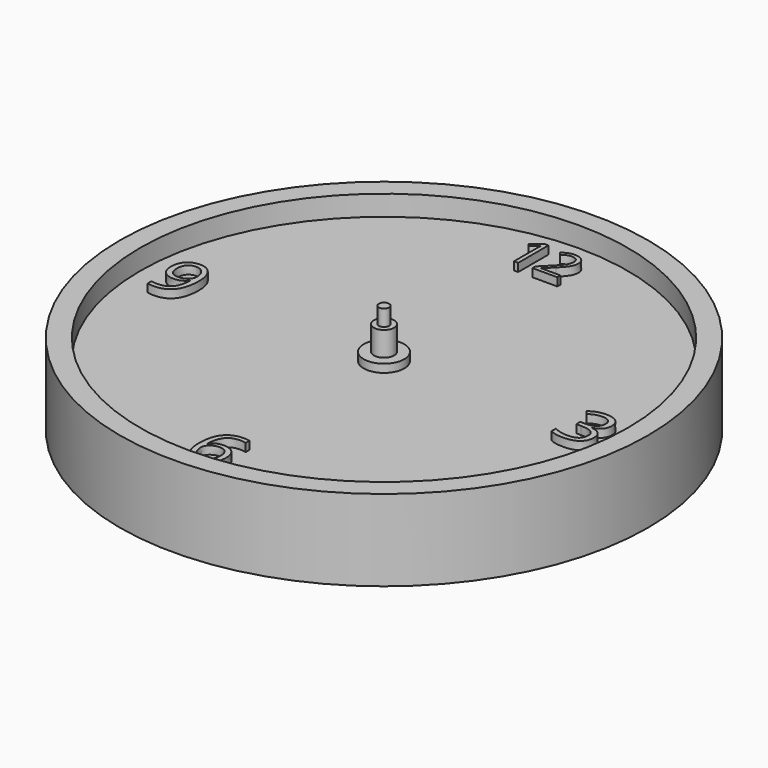
from build123d import *

# Parameters (mm, degrees)
F0_W           = 76.2
F0_H           = 6.35
F3_R           = 6.35
F3_R_2         = 3.175
F3_TEXT_SIZE   = 16.49797023
F3_TEXT_SIZE_2 = 21.9735063531
F3_TEXT_SIZE_3 = 21.605528974
F3_TEXT_SIZE_4 = 21.7850442241
F4_DEPTH       = 2.54
F3_R_3         = 1.5875
F5_DEPTH       = 6.35
F6_DEPTH       = 10.16
F6_DEPTH_BACK  = 12.7
F7_DEPTH       = 15.24
F7_DEPTH_BACK  = 25.4
F8_R           = 3.175
F9_DEPTH       = 6.35
F8_R_2         = 1.8294732505


# Not quite as in the source:
# - Text() gives the source's letters only with a copy of the font that has no kerning and outlines rounded to 1/6400 em; it was checked with that copy


with BuildPart() as f1:
    # F0 (on Front) → F1 (revolve)
    with BuildSketch(Plane.XZ):
        with Locations((-38.1, 3.175)):
            Rectangle(F0_W, F0_H)
    revolve(axis=Axis((0, 0, 3.175), (0, 0, 1)))

    # F3 (on face) → F5 (cut)
    with BuildSketch(Plane.XY.offset(6.35)):
        Circle(F3_R_2)
        Circle(F3_R_3, mode=Mode.SUBTRACT)
        Circle(F3_R_3)
    extrude(amount=-F5_DEPTH, mode=Mode.SUBTRACT)


with BuildPart() as f2:
    # F0 (on Front) → F2 (revolve)
    with BuildSketch(Plane.XZ):
        Polygon((-76.2, -12.7), (-76.2, 0), (-76.2, 6.35), (-76.2, 12.7), (-82.55, 12.7), (-82.55, -12.7), align=None)
    revolve(axis=Axis((0, 0, 3.175), (0, 0, 1)))


with BuildPart() as f4:
    # F3 (on face) → F4 (new body)
    with BuildSketch(Plane.XY.offset(6.35)):
        Circle(F3_R)
        Circle(F3_R_2, mode=Mode.SUBTRACT)
        with Locations((-9.525, 57.15)):
            Text('12', F3_TEXT_SIZE, font='Open Sans', text_align=(TextAlign.LEFT, TextAlign.BOTTOM))
        with Locations((57.15, -7.9104622871)):
            Text('3', F3_TEXT_SIZE_2, font='Open Sans', text_align=(TextAlign.LEFT, TextAlign.BOTTOM))
        with Locations((-6.35, -72.7059808612)):
            Text('6', F3_TEXT_SIZE_3, font='Open Sans', text_align=(TextAlign.LEFT, TextAlign.BOTTOM))
        with Locations((-69.85, -7.8426159207)):
            Text('9', F3_TEXT_SIZE_4, font='Open Sans', text_align=(TextAlign.LEFT, TextAlign.BOTTOM))
    extrude(amount=F4_DEPTH)


with BuildPart() as f6:
    # F3 (on face) → F6 (new body, two sides)
    with BuildSketch(Plane.XY.offset(6.35)) as f6_sk:
        Circle(F3_R_2)
        Circle(F3_R_3, mode=Mode.SUBTRACT)
    extrude(amount=F6_DEPTH)
    extrude(f6_sk.sketch, amount=-F6_DEPTH_BACK)


with BuildPart() as f7:
    # F3 (on face) → F7 (new body, two sides)
    with BuildSketch(Plane.XY.offset(6.35)) as f7_sk:
        Circle(F3_R_3)
    extrude(amount=F7_DEPTH)
    extrude(f7_sk.sketch, amount=-F7_DEPTH_BACK)


with BuildPart() as f9:
    # F8 (on face) → F9 (new body)
    with BuildSketch(Plane(origin=(0, 0, -19.05), x_dir=(1, 0, 0), z_dir=(0, 0, -1))):
        with BuildLine():
            ThreePointArc((38.0743797192, -1.397), (38.0935943913, -0.6986174559), (38.1, 0))
            ThreePointArc((38.1, 0), (38.0935943913, 0.6986174559), (38.0743797192, 1.397))
            ThreePointArc((38.0743797192, 1.397), (38.0477852741, 1.9939999329), (38.0118305465, 2.5905093141))
            ThreePointArc((38.0118305465, 2.5905093141), (37.8912842135, 3.9825344505), (37.7197780201, 5.3692034897))
            ThreePointArc((37.7197780201, 5.3692034897), (37.6309257767, 5.960153118), (37.5328158038, 6.549636466))
            ThreePointArc((37.5328158038, 6.549636466), (37.267423588, 7.9214354202), (36.9519105397, 9.2825808625))
            ThreePointArc((36.9519105397, 9.2825808625), (36.8017739816, 9.8610056184), (36.642583677, 10.4370044302))
            ThreePointArc((36.642583677, 10.4370044302), (36.2352532708, 11.7735474857), (35.7791901947, 13.0942563368))
            ThreePointArc((35.7791901947, 13.0942563368), (35.5694142495, 13.6538188777), (35.3508877354, 14.2100223898))
            ThreePointArc((35.3508877354, 14.2100223898), (34.8060819362, 15.4966661012), (34.2144655546, 16.7624683985))
            ThreePointArc((34.2144655546, 16.7624683985), (33.9473485716, 17.2970380401), (33.6718800701, 17.8273523705))
            ThreePointArc((33.6718800701, 17.8273523705), (32.9955678842, 19.05), (32.2748800701, 20.2470273487))
            ThreePointArc((32.2748800701, 20.2470273487), (31.9533486387, 20.7507472341), (31.6239562406, 21.249362148))
            ThreePointArc((31.6239562406, 21.249362148), (30.8235474857, 22.3946181123), (29.9816842456, 23.5097556303))
            ThreePointArc((29.9816842456, 23.5097556303), (29.6092611315, 23.977106899), (29.2295537287, 24.438559467))
            ThreePointArc((29.2295537287, 24.438559467), (28.3138178507, 25.4938761023), (27.3600028145, 26.5149061094))
            ThreePointArc((27.3600028145, 26.5149061094), (26.9407683632, 26.9407683632), (26.5149061094, 27.3600028145))
            ThreePointArc((26.5149061094, 27.3600028145), (25.4938761023, 28.3138178507), (24.438559467, 29.2295537287))
            ThreePointArc((24.438559467, 29.2295537287), (23.977106899, 29.6092611315), (23.5097556303, 29.9816842456))
            ThreePointArc((23.5097556303, 29.9816842456), (22.3946181123, 30.8235474857), (21.249362148, 31.6239562406))
            ThreePointArc((21.249362148, 31.6239562406), (20.7507472341, 31.9533486387), (20.2470273487, 32.2748800701))
            ThreePointArc((20.2470273487, 32.2748800701), (19.05, 32.9955678842), (17.8273523705, 33.6718800701))
            ThreePointArc((17.8273523705, 33.6718800701), (17.2970380401, 33.9473485716), (16.7624683985, 34.2144655546))
            ThreePointArc((16.7624683985, 34.2144655546), (15.4966661012, 34.8060819362), (14.2100223898, 35.3508877354))
            ThreePointArc((14.2100223898, 35.3508877354), (13.6538188777, 35.5694142495), (13.0942563368, 35.7791901947))
            ThreePointArc((13.0942563368, 35.7791901947), (11.7735474857, 36.2352532708), (10.4370044302, 36.642583677))
            ThreePointArc((10.4370044302, 36.642583677), (9.8610056184, 36.8017739816), (9.2825808625, 36.9519105397))
            ThreePointArc((9.2825808625, 36.9519105397), (7.9214354202, 37.267423588), (6.549636466, 37.5328158038))
            ThreePointArc((6.549636466, 37.5328158038), (5.960153118, 37.6309257767), (5.3692034897, 37.7197780201))
            ThreePointArc((5.3692034897, 37.7197780201), (3.9825344505, 37.8912842135), (2.5905093141, 38.0118305465))
            ThreePointArc((2.5905093141, 38.0118305465), (1.9939999329, 38.0477852741), (1.397, 38.0743797192))
            ThreePointArc((1.397, 38.0743797192), (0, 38.1), (-1.397, 38.0743797192))
            ThreePointArc((-1.397, 38.0743797192), (-1.9939999329, 38.0477852741), (-2.5905093141, 38.0118305465))
            ThreePointArc((-2.5905093141, 38.0118305465), (-3.9825344505, 37.8912842135), (-5.3692034897, 37.7197780201))
            ThreePointArc((-5.3692034897, 37.7197780201), (-5.960153118, 37.6309257767), (-6.549636466, 37.5328158038))
            ThreePointArc((-6.549636466, 37.5328158038), (-7.9214354202, 37.267423588), (-9.2825808625, 36.9519105397))
            ThreePointArc((-9.2825808625, 36.9519105397), (-9.8610056184, 36.8017739816), (-10.4370044302, 36.642583677))
            ThreePointArc((-10.4370044302, 36.642583677), (-11.7735474857, 36.2352532708), (-13.0942563368, 35.7791901947))
            ThreePointArc((-13.0942563368, 35.7791901947), (-13.6538188777, 35.5694142495), (-14.2100223898, 35.3508877354))
            ThreePointArc((-14.2100223898, 35.3508877354), (-15.4966661012, 34.8060819362), (-16.7624683985, 34.2144655546))
            ThreePointArc((-16.7624683985, 34.2144655546), (-17.2970380401, 33.9473485716), (-17.8273523705, 33.6718800701))
            ThreePointArc((-17.8273523705, 33.6718800701), (-19.05, 32.9955678842), (-20.2470273487, 32.2748800701))
            ThreePointArc((-20.2470273487, 32.2748800701), (-20.7507472341, 31.9533486387), (-21.249362148, 31.6239562406))
            ThreePointArc((-21.249362148, 31.6239562406), (-22.3946181123, 30.8235474857), (-23.5097556303, 29.9816842456))
            ThreePointArc((-23.5097556303, 29.9816842456), (-23.977106899, 29.6092611315), (-24.438559467, 29.2295537287))
            ThreePointArc((-24.438559467, 29.2295537287), (-25.4938761023, 28.3138178507), (-26.5149061094, 27.3600028145))
            ThreePointArc((-26.5149061094, 27.3600028145), (-26.9407683632, 26.9407683632), (-27.3600028145, 26.5149061094))
            ThreePointArc((-27.3600028145, 26.5149061094), (-28.3138178507, 25.4938761023), (-29.2295537287, 24.438559467))
            ThreePointArc((-29.2295537287, 24.438559467), (-29.6092611315, 23.977106899), (-29.9816842456, 23.5097556303))
            ThreePointArc((-29.9816842456, 23.5097556303), (-30.8235474857, 22.3946181123), (-31.6239562406, 21.249362148))
            ThreePointArc((-31.6239562406, 21.249362148), (-31.9533486387, 20.7507472341), (-32.2748800701, 20.2470273487))
            ThreePointArc((-32.2748800701, 20.2470273487), (-32.9955678842, 19.05), (-33.6718800701, 17.8273523705))
            ThreePointArc((-33.6718800701, 17.8273523705), (-33.9473485716, 17.2970380401), (-34.2144655546, 16.7624683985))
            ThreePointArc((-34.2144655546, 16.7624683985), (-34.8060819362, 15.4966661012), (-35.3508877354, 14.2100223898))
            ThreePointArc((-35.3508877354, 14.2100223898), (-35.5694142495, 13.6538188777), (-35.7791901947, 13.0942563368))
            ThreePointArc((-35.7791901947, 13.0942563368), (-36.2352532708, 11.7735474857), (-36.642583677, 10.4370044302))
            ThreePointArc((-36.642583677, 10.4370044302), (-36.8017739816, 9.8610056184), (-36.9519105397, 9.2825808625))
            ThreePointArc((-36.9519105397, 9.2825808625), (-37.267423588, 7.9214354202), (-37.5328158038, 6.549636466))
            ThreePointArc((-37.5328158038, 6.549636466), (-37.6309257767, 5.960153118), (-37.7197780201, 5.3692034897))
            ThreePointArc((-37.7197780201, 5.3692034897), (-37.8912842135, 3.9825344505), (-38.0118305465, 2.5905093141))
            ThreePointArc((-38.0118305465, 2.5905093141), (-38.0477852741, 1.9939999329), (-38.0743797192, 1.397))
            ThreePointArc((-38.0743797192, 1.397), (-38.1, 0), (-38.0743797192, -1.397))
            ThreePointArc((-38.0743797192, -1.397), (-38.0477852741, -1.9939999329), (-38.0118305465, -2.5905093141))
            ThreePointArc((-38.0118305465, -2.5905093141), (-37.8912842135, -3.9825344505), (-37.7197780201, -5.3692034897))
            ThreePointArc((-37.7197780201, -5.3692034897), (-37.6309257767, -5.960153118), (-37.5328158038, -6.549636466))
            ThreePointArc((-37.5328158038, -6.549636466), (-37.267423588, -7.9214354202), (-36.9519105397, -9.2825808625))
            ThreePointArc((-36.9519105397, -9.2825808625), (-36.8017739816, -9.8610056184), (-36.642583677, -10.4370044302))
            ThreePointArc((-36.642583677, -10.4370044302), (-36.2352532708, -11.7735474857), (-35.7791901947, -13.0942563368))
            ThreePointArc((-35.7791901947, -13.0942563368), (-35.5694142495, -13.6538188777), (-35.3508877354, -14.2100223898))
            ThreePointArc((-35.3508877354, -14.2100223898), (-34.8060819362, -15.4966661012), (-34.2144655546, -16.7624683985))
            ThreePointArc((-34.2144655546, -16.7624683985), (-33.9473485716, -17.2970380401), (-33.6718800701, -17.8273523705))
            ThreePointArc((-33.6718800701, -17.8273523705), (-32.9955678842, -19.05), (-32.2748800701, -20.2470273487))
            ThreePointArc((-32.2748800701, -20.2470273487), (-31.9533486387, -20.7507472341), (-31.6239562406, -21.249362148))
            ThreePointArc((-31.6239562406, -21.249362148), (-30.8235474857, -22.3946181123), (-29.9816842456, -23.5097556303))
            ThreePointArc((-29.9816842456, -23.5097556303), (-29.6092611315, -23.977106899), (-29.2295537287, -24.438559467))
            ThreePointArc((-29.2295537287, -24.438559467), (-28.3138178507, -25.4938761023), (-27.3600028145, -26.5149061094))
            ThreePointArc((-27.3600028145, -26.5149061094), (-26.9407683632, -26.9407683632), (-26.5149061094, -27.3600028145))
            ThreePointArc((-26.5149061094, -27.3600028145), (-25.4938761023, -28.3138178507), (-24.438559467, -29.2295537287))
            ThreePointArc((-24.438559467, -29.2295537287), (-23.977106899, -29.6092611315), (-23.5097556303, -29.9816842456))
            ThreePointArc((-23.5097556303, -29.9816842456), (-22.3946181123, -30.8235474857), (-21.249362148, -31.6239562406))
            ThreePointArc((-21.249362148, -31.6239562406), (-20.7507472341, -31.9533486387), (-20.2470273487, -32.2748800701))
            ThreePointArc((-20.2470273487, -32.2748800701), (-19.05, -32.9955678842), (-17.8273523705, -33.6718800701))
            ThreePointArc((-17.8273523705, -33.6718800701), (-17.2970380401, -33.9473485716), (-16.7624683985, -34.2144655546))
            ThreePointArc((-16.7624683985, -34.2144655546), (-15.4966661012, -34.8060819362), (-14.2100223898, -35.3508877354))
            ThreePointArc((-14.2100223898, -35.3508877354), (-13.6538188777, -35.5694142495), (-13.0942563368, -35.7791901947))
            ThreePointArc((-13.0942563368, -35.7791901947), (-11.7735474857, -36.2352532708), (-10.4370044302, -36.642583677))
            ThreePointArc((-10.4370044302, -36.642583677), (-9.8610056184, -36.8017739816), (-9.2825808625, -36.9519105397))
            ThreePointArc((-9.2825808625, -36.9519105397), (-7.9214354202, -37.267423588), (-6.549636466, -37.5328158038))
            ThreePointArc((-6.549636466, -37.5328158038), (-5.960153118, -37.6309257767), (-5.3692034897, -37.7197780201))
            ThreePointArc((-5.3692034897, -37.7197780201), (-3.9825344505, -37.8912842135), (-2.5905093141, -38.0118305465))
            ThreePointArc((-2.5905093141, -38.0118305465), (-1.9939999329, -38.0477852741), (-1.397, -38.0743797192))
            ThreePointArc((-1.397, -38.0743797192), (0, -38.1), (1.397, -38.0743797192))
            ThreePointArc((1.397, -38.0743797192), (1.9939999329, -38.0477852741), (2.5905093141, -38.0118305465))
            ThreePointArc((2.5905093141, -38.0118305465), (3.9825344505, -37.8912842135), (5.3692034897, -37.7197780201))
            ThreePointArc((5.3692034897, -37.7197780201), (5.960153118, -37.6309257767), (6.549636466, -37.5328158038))
            ThreePointArc((6.549636466, -37.5328158038), (7.9214354202, -37.267423588), (9.2825808625, -36.9519105397))
            ThreePointArc((9.2825808625, -36.9519105397), (9.8610056184, -36.8017739816), (10.4370044302, -36.642583677))
            ThreePointArc((10.4370044302, -36.642583677), (11.7735474857, -36.2352532708), (13.0942563368, -35.7791901947))
            ThreePointArc((13.0942563368, -35.7791901947), (13.6538188777, -35.5694142495), (14.2100223898, -35.3508877354))
            ThreePointArc((14.2100223898, -35.3508877354), (15.4966661012, -34.8060819362), (16.7624683985, -34.2144655546))
            ThreePointArc((16.7624683985, -34.2144655546), (17.2970380401, -33.9473485716), (17.8273523705, -33.6718800701))
            ThreePointArc((17.8273523705, -33.6718800701), (19.05, -32.9955678842), (20.2470273487, -32.2748800701))
            ThreePointArc((20.2470273487, -32.2748800701), (20.7507472341, -31.9533486387), (21.249362148, -31.6239562406))
            ThreePointArc((21.249362148, -31.6239562406), (22.3946181123, -30.8235474857), (23.5097556303, -29.9816842456))
            ThreePointArc((23.5097556303, -29.9816842456), (23.977106899, -29.6092611315), (24.438559467, -29.2295537287))
            ThreePointArc((24.438559467, -29.2295537287), (25.4938761023, -28.3138178507), (26.5149061094, -27.3600028145))
            ThreePointArc((26.5149061094, -27.3600028145), (26.9407683632, -26.9407683632), (27.3600028145, -26.5149061094))
            ThreePointArc((27.3600028145, -26.5149061094), (28.3138178507, -25.4938761023), (29.2295537287, -24.438559467))
            ThreePointArc((29.2295537287, -24.438559467), (29.6092611315, -23.977106899), (29.9816842456, -23.5097556303))
            ThreePointArc((29.9816842456, -23.5097556303), (30.8235474857, -22.3946181123), (31.6239562406, -21.249362148))
            ThreePointArc((31.6239562406, -21.249362148), (31.9533486387, -20.7507472341), (32.2748800701, -20.2470273487))
            ThreePointArc((32.2748800701, -20.2470273487), (32.9955678842, -19.05), (33.6718800701, -17.8273523705))
            ThreePointArc((33.6718800701, -17.8273523705), (33.9473485716, -17.2970380401), (34.2144655546, -16.7624683985))
            ThreePointArc((34.2144655546, -16.7624683985), (34.8060819362, -15.4966661012), (35.3508877354, -14.2100223898))
            ThreePointArc((35.3508877354, -14.2100223898), (35.5694142495, -13.6538188777), (35.7791901947, -13.0942563368))
            ThreePointArc((35.7791901947, -13.0942563368), (36.2352532708, -11.7735474857), (36.642583677, -10.4370044302))
            ThreePointArc((36.642583677, -10.4370044302), (36.8017739816, -9.8610056184), (36.9519105397, -9.2825808625))
            ThreePointArc((36.9519105397, -9.2825808625), (37.267423588, -7.9214354202), (37.5328158038, -6.549636466))
            ThreePointArc((37.5328158038, -6.549636466), (37.6309257767, -5.960153118), (37.7197780201, -5.3692034897))
            ThreePointArc((37.7197780201, -5.3692034897), (37.8912842135, -3.9825344505), (38.0118305465, -2.5905093141))
            ThreePointArc((38.0118305465, -2.5905093141), (38.0477852741, -1.9939999329), (38.0743797192, -1.397))
        make_face()
        Circle(F8_R, mode=Mode.SUBTRACT)
        with BuildLine():
            ThreePointArc((38.0743797192, 1.397), (38.0935943913, 0.6986174559), (38.1, 0))
            ThreePointArc((38.1, 0), (38.0935943913, -0.6986174559), (38.0743797192, -1.397))
            Line((38.0743797192, -1.397), (40.4290227388, -0.4445))
            Line((40.4290227388, -0.4445), (40.4290227388, 0.4445))
            Line((40.4290227388, 0.4445), (38.0743797192, 1.397))
        make_face()
        with BuildLine():
            ThreePointArc((37.7197780201, 5.3692034897), (37.8912842135, 3.9825344505), (38.0118305465, 2.5905093141))
            Line((38.0118305465, 2.5905093141), (40.254011224, 3.7839186358))
            Line((40.254011224, 3.7839186358), (40.1610854202, 4.6680486008))
            Line((40.1610854202, 4.6680486008), (37.7197780201, 5.3692034897))
        make_face()
        with BuildLine():
            Line((40.254011224, -3.7839186358), (38.0118305465, -2.5905093141))
            ThreePointArc((38.0118305465, -2.5905093141), (37.8912842135, -3.9825344505), (37.7197780201, -5.3692034897))
            Line((37.7197780201, -5.3692034897), (40.1610854202, -4.6680486008))
            Line((40.1610854202, -4.6680486008), (40.254011224, -3.7839186358))
        make_face()
        with BuildLine():
            ThreePointArc((36.9519105397, 9.2825808625), (37.267423588, 7.9214354202), (37.5328158038, 6.549636466))
            Line((37.5328158038, 6.549636466), (39.6379683386, 7.9708798672))
            Line((39.6379683386, 7.9708798672), (39.4531348454, 8.8404530843))
            Line((39.4531348454, 8.8404530843), (36.9519105397, 9.2825808625))
        make_face()
        with BuildLine():
            Line((39.6379683386, -7.9708798672), (37.5328158038, -6.549636466))
            ThreePointArc((37.5328158038, -6.549636466), (37.267423588, -7.9214354202), (36.9519105397, -9.2825808625))
            Line((36.9519105397, -9.2825808625), (39.4531348454, -8.8404530843))
            Line((39.4531348454, -8.8404530843), (39.6379683386, -7.9708798672))
        make_face()
        with BuildLine():
            ThreePointArc((35.7791901947, 13.0942563368), (36.2352532708, 11.7735474857), (36.642583677, 10.4370044302))
            Line((36.642583677, 10.4370044302), (38.5876435772, 12.0705104708))
            Line((38.5876435772, 12.0705104708), (38.3129274692, 12.9159997138))
            Line((38.3129274692, 12.9159997138), (35.7791901947, 13.0942563368))
        make_face()
        with BuildLine():
            Line((38.5876435772, -12.0705104708), (36.642583677, -10.4370044302))
            ThreePointArc((36.642583677, -10.4370044302), (36.2352532708, -11.7735474857), (35.7791901947, -13.0942563368))
            Line((35.7791901947, -13.0942563368), (38.3129274692, -12.9159997138))
            Line((38.3129274692, -12.9159997138), (38.5876435772, -12.0705104708))
        make_face()
        with BuildLine():
            ThreePointArc((34.2144655546, 16.7624683985), (34.8060819362, 15.4966661012), (35.3508877354, 14.2100223898))
            Line((35.3508877354, 14.2100223898), (37.1145445178, 16.0378940357))
            Line((37.1145445178, 16.0378940357), (36.7529556421, 16.8500359475))
            Line((36.7529556421, 16.8500359475), (34.2144655546, 16.7624683985))
        make_face()
        with BuildLine():
            Line((37.1145445178, -16.0378940357), (35.3508877354, -14.2100223898))
            ThreePointArc((35.3508877354, -14.2100223898), (34.8060819362, -15.4966661012), (34.2144655546, -16.7624683985))
            Line((34.2144655546, -16.7624683985), (36.7529556421, -16.8500359475))
            Line((36.7529556421, -16.8500359475), (37.1145445178, -16.0378940357))
        make_face()
        with BuildLine():
            ThreePointArc((32.2748800701, 20.2470273487), (32.9955678842, 19.05), (33.6718800701, 17.8273523705))
            Line((33.6718800701, 17.8273523705), (35.234810742, 19.8295630774))
            Line((35.234810742, 19.8295630774), (34.790310742, 20.5994596614))
            Line((34.790310742, 20.5994596614), (32.2748800701, 20.2470273487))
        make_face()
        with BuildLine():
            Line((35.234810742, -19.8295630774), (33.6718800701, -17.8273523705))
            ThreePointArc((33.6718800701, -17.8273523705), (32.9955678842, -19.05), (32.2748800701, -20.2470273487))
            Line((32.2748800701, -20.2470273487), (34.790310742, -20.5994596614))
            Line((34.790310742, -20.5994596614), (35.234810742, -19.8295630774))
        make_face()
        with BuildLine():
            ThreePointArc((29.9816842456, 23.5097556303), (30.8235474857, 22.3946181123), (31.6239562406, 21.249362148))
            Line((31.6239562406, 21.249362148), (32.9690370063, 23.4039752765))
            Line((32.9690370063, 23.4039752765), (32.446495917, 24.1231913845))
            Line((32.446495917, 24.1231913845), (29.9816842456, 23.5097556303))
        make_face()
        with BuildLine():
            Line((32.9690370063, -23.4039752765), (31.6239562406, -21.249362148))
            ThreePointArc((31.6239562406, -21.249362148), (30.8235474857, -22.3946181123), (29.9816842456, -23.5097556303))
            Line((29.9816842456, -23.5097556303), (32.446495917, -24.1231913845))
            Line((32.446495917, -24.1231913845), (32.9690370063, -23.4039752765))
        make_face()
        with BuildLine():
            ThreePointArc((27.3600028145, 26.5149061094), (28.3138178507, 25.4938761023), (29.2295537287, 24.438559467))
            Line((29.2295537287, 24.438559467), (30.342047602, 26.7219686248))
            Line((30.342047602, 26.7219686248), (29.7471904929, 27.3826243747))
            Line((29.7471904929, 27.3826243747), (27.3600028145, 26.5149061094))
        make_face()
        with BuildLine():
            Line((30.342047602, -26.7219686248), (29.2295537287, -24.438559467))
            ThreePointArc((29.2295537287, -24.438559467), (28.3138178507, -25.4938761023), (27.3600028145, -26.5149061094))
            Line((27.3600028145, -26.5149061094), (29.7471904929, -27.3826243747))
            Line((29.7471904929, -27.3826243747), (30.342047602, -26.7219686248))
        make_face()
        with BuildLine():
            ThreePointArc((24.438559467, 29.2295537287), (25.4938761023, 28.3138178507), (26.5149061094, 27.3600028145))
            Line((26.5149061094, 27.3600028145), (27.3826243747, 29.7471904929))
            Line((27.3826243747, 29.7471904929), (26.7219686248, 30.342047602))
            Line((26.7219686248, 30.342047602), (24.438559467, 29.2295537287))
        make_face()
        with BuildLine():
            Line((27.3826243747, -29.7471904929), (26.5149061094, -27.3600028145))
            ThreePointArc((26.5149061094, -27.3600028145), (25.4938761023, -28.3138178507), (24.438559467, -29.2295537287))
            Line((24.438559467, -29.2295537287), (26.7219686248, -30.342047602))
            Line((26.7219686248, -30.342047602), (27.3826243747, -29.7471904929))
        make_face()
        with BuildLine():
            ThreePointArc((21.249362148, 31.6239562406), (22.3946181123, 30.8235474857), (23.5097556303, 29.9816842456))
            Line((23.5097556303, 29.9816842456), (24.1231913845, 32.446495917))
            Line((24.1231913845, 32.446495917), (23.4039752765, 32.9690370063))
            Line((23.4039752765, 32.9690370063), (21.249362148, 31.6239562406))
        make_face()
        with BuildLine():
            Line((24.1231913845, -32.446495917), (23.5097556303, -29.9816842456))
            ThreePointArc((23.5097556303, -29.9816842456), (22.3946181123, -30.8235474857), (21.249362148, -31.6239562406))
            Line((21.249362148, -31.6239562406), (23.4039752765, -32.9690370063))
            Line((23.4039752765, -32.9690370063), (24.1231913845, -32.446495917))
        make_face()
        with BuildLine():
            ThreePointArc((17.8273523705, 33.6718800701), (19.05, 32.9955678842), (20.2470273487, 32.2748800701))
            Line((20.2470273487, 32.2748800701), (20.5994596614, 34.790310742))
            Line((20.5994596614, 34.790310742), (19.8295630774, 35.234810742))
            Line((19.8295630774, 35.234810742), (17.8273523705, 33.6718800701))
        make_face()
        with BuildLine():
            Line((20.5994596614, -34.790310742), (20.2470273487, -32.2748800701))
            ThreePointArc((20.2470273487, -32.2748800701), (19.05, -32.9955678842), (17.8273523705, -33.6718800701))
            Line((17.8273523705, -33.6718800701), (19.8295630774, -35.234810742))
            Line((19.8295630774, -35.234810742), (20.5994596614, -34.790310742))
        make_face()
        with BuildLine():
            ThreePointArc((14.2100223898, 35.3508877354), (15.4966661012, 34.8060819362), (16.7624683985, 34.2144655546))
            Line((16.7624683985, 34.2144655546), (16.8500359475, 36.7529556421))
            Line((16.8500359475, 36.7529556421), (16.0378940357, 37.1145445178))
            Line((16.0378940357, 37.1145445178), (14.2100223898, 35.3508877354))
        make_face()
        with BuildLine():
            Line((16.8500359475, -36.7529556421), (16.7624683985, -34.2144655546))
            ThreePointArc((16.7624683985, -34.2144655546), (15.4966661012, -34.8060819362), (14.2100223898, -35.3508877354))
            Line((14.2100223898, -35.3508877354), (16.0378940357, -37.1145445178))
            Line((16.0378940357, -37.1145445178), (16.8500359475, -36.7529556421))
        make_face()
        with BuildLine():
            ThreePointArc((10.4370044302, 36.642583677), (11.7735474857, 36.2352532708), (13.0942563368, 35.7791901947))
            Line((13.0942563368, 35.7791901947), (12.9159997138, 38.3129274692))
            Line((12.9159997138, 38.3129274692), (12.0705104708, 38.5876435772))
            Line((12.0705104708, 38.5876435772), (10.4370044302, 36.642583677))
        make_face()
        with BuildLine():
            Line((12.9159997138, -38.3129274692), (13.0942563368, -35.7791901947))
            ThreePointArc((13.0942563368, -35.7791901947), (11.7735474857, -36.2352532708), (10.4370044302, -36.642583677))
            Line((10.4370044302, -36.642583677), (12.0705104708, -38.5876435772))
            Line((12.0705104708, -38.5876435772), (12.9159997138, -38.3129274692))
        make_face()
        with BuildLine():
            ThreePointArc((6.549636466, 37.5328158038), (7.9214354202, 37.267423588), (9.2825808625, 36.9519105397))
            Line((9.2825808625, 36.9519105397), (8.8404530843, 39.4531348454))
            Line((8.8404530843, 39.4531348454), (7.9708798672, 39.6379683386))
            Line((7.9708798672, 39.6379683386), (6.549636466, 37.5328158038))
        make_face()
        with BuildLine():
            Line((8.8404530843, -39.4531348454), (9.2825808625, -36.9519105397))
            ThreePointArc((9.2825808625, -36.9519105397), (7.9214354202, -37.267423588), (6.549636466, -37.5328158038))
            Line((6.549636466, -37.5328158038), (7.9708798672, -39.6379683386))
            Line((7.9708798672, -39.6379683386), (8.8404530843, -39.4531348454))
        make_face()
        with BuildLine():
            ThreePointArc((2.5905093141, 38.0118305465), (3.9825344505, 37.8912842135), (5.3692034897, 37.7197780201))
            Line((5.3692034897, 37.7197780201), (4.6680486008, 40.1610854202))
            Line((4.6680486008, 40.1610854202), (3.7839186358, 40.254011224))
            Line((3.7839186358, 40.254011224), (2.5905093141, 38.0118305465))
        make_face()
        with BuildLine():
            Line((4.6680486008, -40.1610854202), (5.3692034897, -37.7197780201))
            ThreePointArc((5.3692034897, -37.7197780201), (3.9825344505, -37.8912842135), (2.5905093141, -38.0118305465))
            Line((2.5905093141, -38.0118305465), (3.7839186358, -40.254011224))
            Line((3.7839186358, -40.254011224), (4.6680486008, -40.1610854202))
        make_face()
        with BuildLine():
            ThreePointArc((-1.397, 38.0743797192), (0, 38.1), (1.397, 38.0743797192))
            Line((1.397, 38.0743797192), (0.4445, 40.4290227388))
            Line((0.4445, 40.4290227388), (-0.4445, 40.4290227388))
            Line((-0.4445, 40.4290227388), (-1.397, 38.0743797192))
        make_face()
        with BuildLine():
            Line((0.4445, -40.4290227388), (1.397, -38.0743797192))
            ThreePointArc((1.397, -38.0743797192), (0, -38.1), (-1.397, -38.0743797192))
            Line((-1.397, -38.0743797192), (-0.4445, -40.4290227388))
            Line((-0.4445, -40.4290227388), (0.4445, -40.4290227388))
        make_face()
        with BuildLine():
            ThreePointArc((-5.3692034897, 37.7197780201), (-3.9825344505, 37.8912842135), (-2.5905093141, 38.0118305465))
            Line((-2.5905093141, 38.0118305465), (-3.7839186358, 40.254011224))
            Line((-3.7839186358, 40.254011224), (-4.6680486008, 40.1610854202))
            Line((-4.6680486008, 40.1610854202), (-5.3692034897, 37.7197780201))
        make_face()
        with BuildLine():
            Line((-3.7839186358, -40.254011224), (-2.5905093141, -38.0118305465))
            ThreePointArc((-2.5905093141, -38.0118305465), (-3.9825344505, -37.8912842135), (-5.3692034897, -37.7197780201))
            Line((-5.3692034897, -37.7197780201), (-4.6680486008, -40.1610854202))
            Line((-4.6680486008, -40.1610854202), (-3.7839186358, -40.254011224))
        make_face()
        with BuildLine():
            ThreePointArc((-9.2825808625, 36.9519105397), (-7.9214354202, 37.267423588), (-6.549636466, 37.5328158038))
            Line((-6.549636466, 37.5328158038), (-7.9708798672, 39.6379683386))
            Line((-7.9708798672, 39.6379683386), (-8.8404530843, 39.4531348454))
            Line((-8.8404530843, 39.4531348454), (-9.2825808625, 36.9519105397))
        make_face()
        with BuildLine():
            Line((-7.9708798672, -39.6379683386), (-6.549636466, -37.5328158038))
            ThreePointArc((-6.549636466, -37.5328158038), (-7.9214354202, -37.267423588), (-9.2825808625, -36.9519105397))
            Line((-9.2825808625, -36.9519105397), (-8.8404530843, -39.4531348454))
            Line((-8.8404530843, -39.4531348454), (-7.9708798672, -39.6379683386))
        make_face()
        with BuildLine():
            ThreePointArc((-13.0942563368, 35.7791901947), (-11.7735474857, 36.2352532708), (-10.4370044302, 36.642583677))
            Line((-10.4370044302, 36.642583677), (-12.0705104708, 38.5876435772))
            Line((-12.0705104708, 38.5876435772), (-12.9159997138, 38.3129274692))
            Line((-12.9159997138, 38.3129274692), (-13.0942563368, 35.7791901947))
        make_face()
        with BuildLine():
            Line((-12.0705104708, -38.5876435772), (-10.4370044302, -36.642583677))
            ThreePointArc((-10.4370044302, -36.642583677), (-11.7735474857, -36.2352532708), (-13.0942563368, -35.7791901947))
            Line((-13.0942563368, -35.7791901947), (-12.9159997138, -38.3129274692))
            Line((-12.9159997138, -38.3129274692), (-12.0705104708, -38.5876435772))
        make_face()
        with BuildLine():
            ThreePointArc((-16.7624683985, 34.2144655546), (-15.4966661012, 34.8060819362), (-14.2100223898, 35.3508877354))
            Line((-14.2100223898, 35.3508877354), (-16.0378940357, 37.1145445178))
            Line((-16.0378940357, 37.1145445178), (-16.8500359475, 36.7529556421))
            Line((-16.8500359475, 36.7529556421), (-16.7624683985, 34.2144655546))
        make_face()
        with BuildLine():
            Line((-16.0378940357, -37.1145445178), (-14.2100223898, -35.3508877354))
            ThreePointArc((-14.2100223898, -35.3508877354), (-15.4966661012, -34.8060819362), (-16.7624683985, -34.2144655546))
            Line((-16.7624683985, -34.2144655546), (-16.8500359475, -36.7529556421))
            Line((-16.8500359475, -36.7529556421), (-16.0378940357, -37.1145445178))
        make_face()
        with BuildLine():
            ThreePointArc((-20.2470273487, 32.2748800701), (-19.05, 32.9955678842), (-17.8273523705, 33.6718800701))
            Line((-17.8273523705, 33.6718800701), (-19.8295630774, 35.234810742))
            Line((-19.8295630774, 35.234810742), (-20.5994596614, 34.790310742))
            Line((-20.5994596614, 34.790310742), (-20.2470273487, 32.2748800701))
        make_face()
        with BuildLine():
            Line((-19.8295630774, -35.234810742), (-17.8273523705, -33.6718800701))
            ThreePointArc((-17.8273523705, -33.6718800701), (-19.05, -32.9955678842), (-20.2470273487, -32.2748800701))
            Line((-20.2470273487, -32.2748800701), (-20.5994596614, -34.790310742))
            Line((-20.5994596614, -34.790310742), (-19.8295630774, -35.234810742))
        make_face()
        with BuildLine():
            ThreePointArc((-23.5097556303, 29.9816842456), (-22.3946181123, 30.8235474857), (-21.249362148, 31.6239562406))
            Line((-21.249362148, 31.6239562406), (-23.4039752765, 32.9690370063))
            Line((-23.4039752765, 32.9690370063), (-24.1231913845, 32.446495917))
            Line((-24.1231913845, 32.446495917), (-23.5097556303, 29.9816842456))
        make_face()
        with BuildLine():
            Line((-23.4039752765, -32.9690370063), (-21.249362148, -31.6239562406))
            ThreePointArc((-21.249362148, -31.6239562406), (-22.3946181123, -30.8235474857), (-23.5097556303, -29.9816842456))
            Line((-23.5097556303, -29.9816842456), (-24.1231913845, -32.446495917))
            Line((-24.1231913845, -32.446495917), (-23.4039752765, -32.9690370063))
        make_face()
        with BuildLine():
            ThreePointArc((-26.5149061094, 27.3600028145), (-25.4938761023, 28.3138178507), (-24.438559467, 29.2295537287))
            Line((-24.438559467, 29.2295537287), (-26.7219686248, 30.342047602))
            Line((-26.7219686248, 30.342047602), (-27.3826243747, 29.7471904929))
            Line((-27.3826243747, 29.7471904929), (-26.5149061094, 27.3600028145))
        make_face()
        with BuildLine():
            Line((-26.7219686248, -30.342047602), (-24.438559467, -29.2295537287))
            ThreePointArc((-24.438559467, -29.2295537287), (-25.4938761023, -28.3138178507), (-26.5149061094, -27.3600028145))
            Line((-26.5149061094, -27.3600028145), (-27.3826243747, -29.7471904929))
            Line((-27.3826243747, -29.7471904929), (-26.7219686248, -30.342047602))
        make_face()
        with BuildLine():
            ThreePointArc((-29.2295537287, 24.438559467), (-28.3138178507, 25.4938761023), (-27.3600028145, 26.5149061094))
            Line((-27.3600028145, 26.5149061094), (-29.7471904929, 27.3826243747))
            Line((-29.7471904929, 27.3826243747), (-30.342047602, 26.7219686248))
            Line((-30.342047602, 26.7219686248), (-29.2295537287, 24.438559467))
        make_face()
        with BuildLine():
            Line((-29.7471904929, -27.3826243747), (-27.3600028145, -26.5149061094))
            ThreePointArc((-27.3600028145, -26.5149061094), (-28.3138178507, -25.4938761023), (-29.2295537287, -24.438559467))
            Line((-29.2295537287, -24.438559467), (-30.342047602, -26.7219686248))
            Line((-30.342047602, -26.7219686248), (-29.7471904929, -27.3826243747))
        make_face()
        with BuildLine():
            ThreePointArc((-31.6239562406, 21.249362148), (-30.8235474857, 22.3946181123), (-29.9816842456, 23.5097556303))
            Line((-29.9816842456, 23.5097556303), (-32.446495917, 24.1231913845))
            Line((-32.446495917, 24.1231913845), (-32.9690370063, 23.4039752765))
            Line((-32.9690370063, 23.4039752765), (-31.6239562406, 21.249362148))
        make_face()
        with BuildLine():
            Line((-32.446495917, -24.1231913845), (-29.9816842456, -23.5097556303))
            ThreePointArc((-29.9816842456, -23.5097556303), (-30.8235474857, -22.3946181123), (-31.6239562406, -21.249362148))
            Line((-31.6239562406, -21.249362148), (-32.9690370063, -23.4039752765))
            Line((-32.9690370063, -23.4039752765), (-32.446495917, -24.1231913845))
        make_face()
        with BuildLine():
            ThreePointArc((-33.6718800701, 17.8273523705), (-32.9955678842, 19.05), (-32.2748800701, 20.2470273487))
            Line((-32.2748800701, 20.2470273487), (-34.790310742, 20.5994596614))
            Line((-34.790310742, 20.5994596614), (-35.234810742, 19.8295630774))
            Line((-35.234810742, 19.8295630774), (-33.6718800701, 17.8273523705))
        make_face()
        with BuildLine():
            Line((-34.790310742, -20.5994596614), (-32.2748800701, -20.2470273487))
            ThreePointArc((-32.2748800701, -20.2470273487), (-32.9955678842, -19.05), (-33.6718800701, -17.8273523705))
            Line((-33.6718800701, -17.8273523705), (-35.234810742, -19.8295630774))
            Line((-35.234810742, -19.8295630774), (-34.790310742, -20.5994596614))
        make_face()
        with BuildLine():
            ThreePointArc((-35.3508877354, 14.2100223898), (-34.8060819362, 15.4966661012), (-34.2144655546, 16.7624683985))
            Line((-34.2144655546, 16.7624683985), (-36.7529556421, 16.8500359475))
            Line((-36.7529556421, 16.8500359475), (-37.1145445178, 16.0378940357))
            Line((-37.1145445178, 16.0378940357), (-35.3508877354, 14.2100223898))
        make_face()
        with BuildLine():
            Line((-36.7529556421, -16.8500359475), (-34.2144655546, -16.7624683985))
            ThreePointArc((-34.2144655546, -16.7624683985), (-34.8060819362, -15.4966661012), (-35.3508877354, -14.2100223898))
            Line((-35.3508877354, -14.2100223898), (-37.1145445178, -16.0378940357))
            Line((-37.1145445178, -16.0378940357), (-36.7529556421, -16.8500359475))
        make_face()
        with BuildLine():
            ThreePointArc((-36.642583677, 10.4370044302), (-36.2352532708, 11.7735474857), (-35.7791901947, 13.0942563368))
            Line((-35.7791901947, 13.0942563368), (-38.3129274692, 12.9159997138))
            Line((-38.3129274692, 12.9159997138), (-38.5876435772, 12.0705104708))
            Line((-38.5876435772, 12.0705104708), (-36.642583677, 10.4370044302))
        make_face()
        with BuildLine():
            Line((-38.3129274692, -12.9159997138), (-35.7791901947, -13.0942563368))
            ThreePointArc((-35.7791901947, -13.0942563368), (-36.2352532708, -11.7735474857), (-36.642583677, -10.4370044302))
            Line((-36.642583677, -10.4370044302), (-38.5876435772, -12.0705104708))
            Line((-38.5876435772, -12.0705104708), (-38.3129274692, -12.9159997138))
        make_face()
        with BuildLine():
            ThreePointArc((-37.5328158038, 6.549636466), (-37.267423588, 7.9214354202), (-36.9519105397, 9.2825808625))
            Line((-36.9519105397, 9.2825808625), (-39.4531348454, 8.8404530843))
            Line((-39.4531348454, 8.8404530843), (-39.6379683386, 7.9708798672))
            Line((-39.6379683386, 7.9708798672), (-37.5328158038, 6.549636466))
        make_face()
        with BuildLine():
            Line((-39.4531348454, -8.8404530843), (-36.9519105397, -9.2825808625))
            ThreePointArc((-36.9519105397, -9.2825808625), (-37.267423588, -7.9214354202), (-37.5328158038, -6.549636466))
            Line((-37.5328158038, -6.549636466), (-39.6379683386, -7.9708798672))
            Line((-39.6379683386, -7.9708798672), (-39.4531348454, -8.8404530843))
        make_face()
        with BuildLine():
            ThreePointArc((-38.0118305465, 2.5905093141), (-37.8912842135, 3.9825344505), (-37.7197780201, 5.3692034897))
            Line((-37.7197780201, 5.3692034897), (-40.1610854202, 4.6680486008))
            Line((-40.1610854202, 4.6680486008), (-40.254011224, 3.7839186358))
            Line((-40.254011224, 3.7839186358), (-38.0118305465, 2.5905093141))
        make_face()
        with BuildLine():
            Line((-40.1610854202, -4.6680486008), (-37.7197780201, -5.3692034897))
            ThreePointArc((-37.7197780201, -5.3692034897), (-37.8912842135, -3.9825344505), (-38.0118305465, -2.5905093141))
            Line((-38.0118305465, -2.5905093141), (-40.254011224, -3.7839186358))
            Line((-40.254011224, -3.7839186358), (-40.1610854202, -4.6680486008))
        make_face()
        with BuildLine():
            ThreePointArc((-38.0743797192, -1.397), (-38.1, 0), (-38.0743797192, 1.397))
            Line((-38.0743797192, 1.397), (-40.4290227388, 0.4445))
            Line((-40.4290227388, 0.4445), (-40.4290227388, -0.4445))
            Line((-40.4290227388, -0.4445), (-38.0743797192, -1.397))
        make_face()
    extrude(amount=F9_DEPTH)


with BuildPart() as f9b:
    # F8 (on face) → F9, piece 2 (new body)
    with BuildSketch(Plane(origin=(0, 0, -19.05), x_dir=(1, 0, 0), z_dir=(0, 0, -1))):
        with BuildLine():
            ThreePointArc((62.039617677, -1.0989587588), (62.1864247511, -0.5581726544), (62.2358738736, 0))
            ThreePointArc((62.2358738736, 0), (62.1864247511, 0.5581726544), (62.039617677, 1.0989587588))
            ThreePointArc((62.039617677, 1.0989587588), (61.6295028307, 1.866218176), (61.0265282195, 2.493356772))
            ThreePointArc((61.0265282195, 2.493356772), (60.0420028307, 3.0196044392), (58.936184442, 3.1725506372))
            ThreePointArc((58.936184442, 3.1725506372), (58.0797449164, 3.0196044392), (57.2969712661, 2.63993799))
            ThreePointArc((57.2969712661, 2.63993799), (56.4922449164, 1.866218176), (56.0050677634, 0.861785366))
            ThreePointArc((56.0050677634, 0.861785366), (55.8858738736, 0), (56.0050677634, -0.861785366))
            ThreePointArc((56.0050677634, -0.861785366), (56.4922449164, -1.866218176), (57.2969712661, -2.63993799))
            ThreePointArc((57.2969712661, -2.63993799), (58.0797449164, -3.0196044392), (58.936184442, -3.1725506372))
            ThreePointArc((58.936184442, -3.1725506372), (60.0420028307, -3.0196044392), (61.0265282195, -2.493356772))
            ThreePointArc((61.0265282195, -2.493356772), (61.6295028307, -1.866218176), (62.039617677, -1.0989587588))
        make_face()
        with Locations((59.0608738736, 0)):
            Circle(F8_R_2, mode=Mode.SUBTRACT)
        with BuildLine():
            ThreePointArc((62.039617677, 1.0989587588), (62.1864247511, 0.5581726544), (62.2358738736, 0))
            ThreePointArc((62.2358738736, 0), (62.1864247511, -0.5581726544), (62.039617677, -1.0989587588))
            Line((62.039617677, -1.0989587588), (64.4938555899, -0.4445))
            Line((64.4938555899, -0.4445), (64.4938555899, 0.4445))
            Line((64.4938555899, 0.4445), (62.039617677, 1.0989587588))
        make_face()
        with BuildLine():
            ThreePointArc((58.936184442, 3.1725506372), (60.0420028307, 3.0196044392), (61.0265282195, 2.493356772))
            Line((61.0265282195, 2.493356772), (61.1625021755, 5.0297146102))
            Line((61.1625021755, 5.0297146102), (60.3170129325, 5.3044307182))
            Line((60.3170129325, 5.3044307182), (58.936184442, 3.1725506372))
        make_face()
        with BuildLine():
            Line((61.1625021755, -5.0297146102), (61.0265282195, -2.493356772))
            ThreePointArc((61.0265282195, -2.493356772), (60.0420028307, -3.0196044392), (58.936184442, -3.1725506372))
            Line((58.936184442, -3.1725506372), (60.3170129325, -5.3044307182))
            Line((60.3170129325, -5.3044307182), (61.1625021755, -5.0297146102))
        make_face()
        with BuildLine():
            ThreePointArc((56.0050677634, 0.861785366), (56.4922449164, 1.866218176), (57.2969712661, 2.63993799))
            Line((57.2969712661, 2.63993799), (54.9267698796, 3.5530345828))
            Line((54.9267698796, 3.5530345828), (54.4042287903, 2.8338184748))
            Line((54.4042287903, 2.8338184748), (56.0050677634, 0.861785366))
        make_face()
        with BuildLine():
            Line((54.9267698796, -3.5530345828), (57.2969712661, -2.63993799))
            ThreePointArc((57.2969712661, -2.63993799), (56.4922449164, -1.866218176), (56.0050677634, -0.861785366))
            Line((56.0050677634, -0.861785366), (54.4042287903, -2.8338184748))
            Line((54.4042287903, -2.8338184748), (54.9267698796, -3.5530345828))
        make_face()
    extrude(amount=F9_DEPTH)


solid = Compound([f1.part, f2.part, f4.part, f6.part, f7.part, f9.part, f9b.part])
